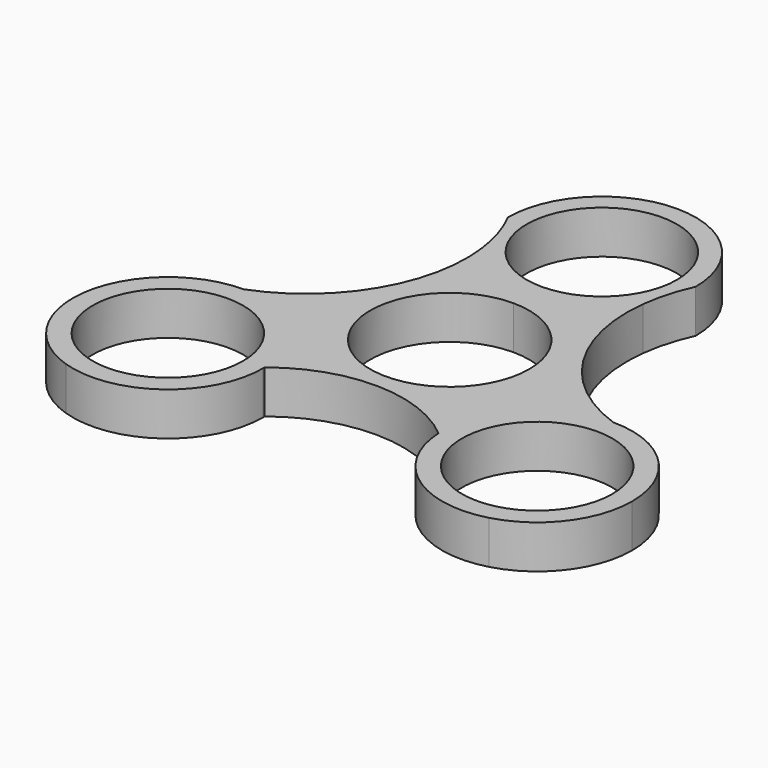
from build123d import *

# Parameters (mm, degrees)
F0_R     = 11.049
F1_DEPTH = 6.35


with BuildPart() as f1:
    # F0 (on Top) → F1 (new body)
    with BuildSketch(Plane.XY):
        with BuildLine():
            ThreePointArc((-11.3469625039, 20.0920200438), (-14.4854082565, 4.9914875059), (-26.2741162088, -4.9534755149))
            ThreePointArc((-26.2741162088, -4.9534755149), (-16.5077935225, -8.934489521), (-12.3076651672, -18.6086020451))
            ThreePointArc((-12.3076651672, -18.6086020451), (0.649772882, -14.1418626943), (13.4943491716, -18.9234755149))
            ThreePointArc((13.4943491716, -18.9234755149), (17.3328597235, -8.6100846058), (27.4479022012, -4.2757898563))
            ThreePointArc((27.4479022012, -4.2757898563), (15.2201160848, 5.4859259906), (11.7737009685, 20.7480383092))
            ThreePointArc((11.7737009685, 20.7480383092), (6.7498223767, 15.9073674809), (0, 14.1434661071))
            ThreePointArc((0, 14.1434661071), (-6.4058342939, 15.720767845), (-11.3469625039, 20.0920200438))
        make_face()
        with BuildLine():
            ThreePointArc((13.97, 0), (-9.8782817332, -9.8782817332), (0, 13.97))
            ThreePointArc((0, 13.97), (9.8782817332, 9.8782817332), (13.97, 0))
        make_face(mode=Mode.SUBTRACT)
        with BuildLine():
            ThreePointArc((13.97, 0), (9.8782817332, 9.8782817332), (0, 13.97))
            ThreePointArc((0, 13.97), (-9.8782817332, -9.8782817332), (13.97, 0))
        make_face()
        with BuildLine():
            ThreePointArc((11.6814433874, 0), (-8.2600278333, -8.2600278333), (0, 11.6814433874))
            ThreePointArc((0, 11.6814433874), (8.2600278333, 8.2600278333), (11.6814433874, 0))
        make_face(mode=Mode.SUBTRACT)
        with BuildLine():
            ThreePointArc((-26.2741162088, -4.9534755149), (-36.1348230129, -9.0276500657), (-40.2440279254, -18.8738103292))
            ThreePointArc((-40.2440279254, -18.8738103292), (-36.068722537, -25.9778704776), (-30.6538718182, -32.1891696469))
            ThreePointArc((-30.6538718182, -32.1891696469), (-18.0895052181, -30.2448289204), (-12.3041162088, -18.9234755149))
            ThreePointArc((-12.3041162088, -18.9234755149), (-12.3050034765, -18.7660287802), (-12.3076651672, -18.6086020451))
            ThreePointArc((-12.3076651672, -18.6086020451), (-16.5077935225, -8.934489521), (-26.2741162088, -4.9534755149))
        make_face()
        with Locations((-26.2741162088, -18.9234755149)):
            Circle(F0_R, mode=Mode.SUBTRACT)
        with BuildLine():
            ThreePointArc((-13.7965338929, 27.94), (-12.227697713, 24.1233976847), (-11.3469625039, 20.0920200438))
            ThreePointArc((-11.3469625039, 20.0920200438), (-6.4058342939, 15.720767845), (0, 14.1434661071))
            ThreePointArc((0, 14.1434661071), (6.7498223767, 15.9073674809), (11.7737009685, 20.7480383092))
            ThreePointArc((11.7737009685, 20.7480383092), (12.4990400343, 24.4244821494), (13.7965338929, 27.94))
            ThreePointArc((13.7965338929, 27.94), (0, 41.7365338929), (-13.7965338929, 27.94))
        make_face()
        with BuildLine():
            ThreePointArc((11.049, 27.94), (7.8128228253, 20.1271771747), (0, 16.891))
            ThreePointArc((0, 16.891), (-7.8128228253, 35.7528228253), (11.049, 27.94))
        make_face(mode=Mode.SUBTRACT)
        with BuildLine():
            ThreePointArc((31.1400760327, -31.7190505009), (37.0174753812, -24.6070928067), (41.3000458498, -16.4349844175))
            ThreePointArc((41.3000458498, -16.4349844175), (36.6637566928, -7.7467934285), (27.4479022012, -4.2757898563))
            ThreePointArc((27.4479022012, -4.2757898563), (17.3328597235, -8.6100846058), (13.4943491716, -18.9234755149))
            ThreePointArc((13.4943491716, -18.9234755149), (19.2469473442, -29.5553097149), (31.1400760327, -31.7190505009))
        make_face()
        with Locations((27.4479022012, -18.2457898563)):
            Circle(F0_R, mode=Mode.SUBTRACT)
        with BuildLine():
            ThreePointArc((41.4179022012, -18.2457898563), (41.3884069763, -17.338471492), (41.3000458498, -16.4349844175))
            ThreePointArc((41.3000458498, -16.4349844175), (37.0174753812, -24.6070928067), (31.1400760327, -31.7190505009))
            ThreePointArc((31.1400760327, -31.7190505009), (38.5551198642, -26.7187241642), (41.4179022012, -18.2457898563))
        make_face()
        with BuildLine():
            ThreePointArc((-30.6538718182, -32.1891696469), (-36.068722537, -25.9778704776), (-40.2440279254, -18.8738103292))
            ThreePointArc((-40.2440279254, -18.8738103292), (-37.6100004347, -27.0879490936), (-30.6538718182, -32.1891696469))
        make_face()
    extrude(amount=F1_DEPTH)


solid = f1.part
